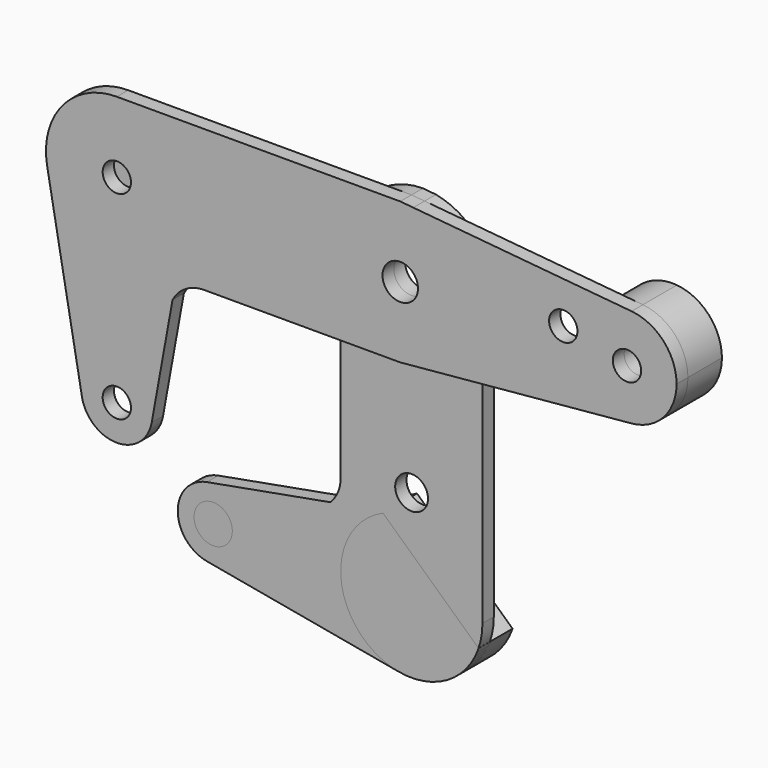
from build123d import *

# Parameters (mm, degrees)
F0_R     = 3.175
F0_R_2   = 3.9751
F2_DEPTH = 3.175
F1_R     = 4.2892452459
F1_R_2   = 3.6765959768
F1_R_3   = 5.1795527056
F3_DEPTH = 3.175
F6_DEPTH = 9.525


with BuildPart() as f2:
    # F0 (on Front) → F2 (new body)
    with BuildSketch(Plane.XZ):
        with BuildLine():
            ThreePointArc((-63.5, 15.875), (-52.2746798487, 11.2253201513), (-47.625, 0))
            ThreePointArc((-47.625, 0), (-62.076859197, -15.8110814069), (-79.1198403471, -2.8348214286))
            Line((-79.1198403471, -2.8348214286), (-71.3099201735, -45.8674107143))
            ThreePointArc((-71.3099201735, -45.8674107143), (-64.2115704015, -36.5444592966), (-55.5625, -44.45))
            ThreePointArc((-55.5625, -44.45), (-55.5944592966, -45.1615704015), (-55.6900798265, -45.8674107143))
            Line((-55.6900798265, -45.8674107143), (-51.0209685693, -20.140650057))
            ThreePointArc((-51.0209685693, -20.140650057), (-48.093941688, -17.0245166153), (-43.976128489, -15.875))
            Line((-43.976128489, -15.875), (0, -15.875))
            ThreePointArc((0, -15.875), (-15.875, 0), (0, 15.875))
            Line((0, 15.875), (-63.5, 15.875))
        make_face()
        with BuildLine():
            Line((51.8269366371, 11.0649472386), (2.9215490166, 15.6038513305))
            ThreePointArc((2.9215490166, 15.6038513305), (12.2146472655, 10.1399219514), (15.875, 0))
            ThreePointArc((15.875, 0), (12.2146472655, -10.1399219514), (2.9215490166, -15.6038513305))
            Line((2.9215490166, -15.6038513305), (51.8269366371, -11.0649472386))
            ThreePointArc((51.8269366371, -11.0649472386), (39.6875, 0), (51.8269366371, 11.0649472386))
        make_face()
        with Locations((36.5252, 3.175)):
            Circle(F0_R, mode=Mode.SUBTRACT)
        with BuildLine():
            Line((2.9215490166, 15.6038513305), (0, 15.875))
            ThreePointArc((0, 15.875), (-15.875, 0), (0, -15.875))
            Line((0, -15.875), (2.9215490166, -15.6038513305))
            ThreePointArc((2.9215490166, -15.6038513305), (12.2146472655, -10.1399219514), (15.875, 0))
            ThreePointArc((15.875, 0), (12.2146472655, 10.1399219514), (2.9215490166, 15.6038513305))
        make_face()
        Circle(F0_R_2, mode=Mode.SUBTRACT)
        with BuildLine():
            ThreePointArc((61.9125, 0), (59.0127793599, 7.4858474093), (51.8269366371, 11.0649472386))
            ThreePointArc((51.8269366371, 11.0649472386), (39.6875, 0), (51.8269366371, -11.0649472386))
            ThreePointArc((51.8269366371, -11.0649472386), (59.0127793599, -7.4858474093), (61.9125, 0))
        make_face()
        with Locations((50.8, 0)):
            Circle(F0_R, mode=Mode.SUBTRACT)
        with BuildLine():
            ThreePointArc((-79.1198403471, -2.8348214286), (-62.076859197, -15.8110814069), (-47.625, 0))
            ThreePointArc((-47.625, 0), (-52.2746798487, 11.2253201513), (-63.5, 15.875))
            ThreePointArc((-63.5, 15.875), (-75.6864353931, 10.1738103683), (-79.1198403471, -2.8348214286))
        make_face()
        with Locations((-63.5, 0)):
            Circle(F0_R, mode=Mode.SUBTRACT)
        with BuildLine():
            ThreePointArc((-55.5625, -44.45), (-64.2115704015, -36.5444592966), (-71.3099201735, -45.8674107143))
            ThreePointArc((-71.3099201735, -45.8674107143), (-63.5, -52.3875), (-55.6900798265, -45.8674107143))
            ThreePointArc((-55.6900798265, -45.8674107143), (-55.5944592966, -45.1615704015), (-55.5625, -44.45))
        make_face()
        with Locations((-63.5, -44.45)):
            Circle(F0_R, mode=Mode.SUBTRACT)
    extrude(amount=F2_DEPTH)


with BuildPart() as f3:
    # F1 (on Front) → F3 (new body)
    with BuildSketch(Plane.XZ):
        with BuildLine():
            ThreePointArc((-45.8674107143, -55.6900798265), (-52.3875, -63.5), (-45.8674107143, -71.3099201735))
            ThreePointArc((-45.8674107143, -71.3099201735), (-39.3630948158, -69.5932176965), (-36.5125, -63.5))
            ThreePointArc((-36.5125, -63.5), (-39.3630948158, -57.4067823035), (-45.8674107143, -55.6900798265))
        make_face()
        with Locations((-44.45, -63.5)):
            Circle(F1_R, mode=Mode.SUBTRACT)
        with BuildLine():
            ThreePointArc((-2.8348214286, -79.1198403471), (-10.1738103683, -51.3135646069), (15.875, -63.5))
            Line((15.875, -63.5), (15.875, 0))
            ThreePointArc((15.875, 0), (0, -15.875), (-15.875, 0))
            Line((-15.875, 0), (-15.875, -45.0455299837))
            ThreePointArc((-15.875, -45.0455299837), (-16.4809135011, -48.0897270637), (-18.2062962849, -50.6699056006))
            Line((-18.2062962849, -50.6699056006), (-45.8674107143, -55.6900798265))
            ThreePointArc((-45.8674107143, -55.6900798265), (-39.3630948158, -57.4067823035), (-36.5125, -63.5))
            ThreePointArc((-36.5125, -63.5), (-39.3630948158, -69.5932176965), (-45.8674107143, -71.3099201735))
            Line((-45.8674107143, -71.3099201735), (-2.8348214286, -79.1198403471))
        make_face()
        with Locations((0, -42.8498)):
            Circle(F1_R_2, mode=Mode.SUBTRACT)
        with BuildLine():
            ThreePointArc((-2.8348214286, -79.1198403471), (10.1738103683, -75.6864353931), (15.875, -63.5))
            ThreePointArc((15.875, -63.5), (-10.1738103683, -51.3135646069), (-2.8348214286, -79.1198403471))
        make_face()
        with Locations((0, -63.5)):
            Circle(F1_R_3, mode=Mode.SUBTRACT)
    extrude(amount=-F3_DEPTH)

    # F0 (on Front) → F3, piece 2 (join)
    with BuildSketch(Plane.XZ):
        with BuildLine():
            Line((2.9215490166, 15.6038513305), (0, 15.875))
            ThreePointArc((0, 15.875), (-15.875, 0), (0, -15.875))
            Line((0, -15.875), (2.9215490166, -15.6038513305))
            ThreePointArc((2.9215490166, -15.6038513305), (12.2146472655, -10.1399219514), (15.875, 0))
            ThreePointArc((15.875, 0), (12.2146472655, 10.1399219514), (2.9215490166, 15.6038513305))
        make_face()
        Circle(F0_R_2, mode=Mode.SUBTRACT)
    extrude(amount=-F3_DEPTH)


with BuildPart() as f6:
    # F4 (on face) → F6 (new body, through all)
    with BuildSketch(Plane.XZ):
        with BuildLine():
            Line((15.0065312392, -68.678768692), (-6.4073053166, -48.9754668378))
            ThreePointArc((-6.4073053166, -48.9754668378), (-15.7646769793, -65.3683106647), (-2.8348214286, -79.1198403471))
            ThreePointArc((-2.8348214286, -79.1198403471), (8.0182058002, -77.2012408469), (15.0065312392, -68.678768692))
        make_face()
    extrude(amount=-F6_DEPTH)


with BuildPart() as f6b:
    # F1 (on Front) → F6, piece 2 (new body, through all)
    with BuildSketch(Plane.XZ):
        with Locations((-44.45, -63.5)):
            Circle(F1_R)
    extrude(amount=-F6_DEPTH)


with BuildPart() as f6c:
    # F0 (on Front) → F6, piece 3 (new body, through all)
    with BuildSketch(Plane.XZ):
        with Locations((-63.5, 0)):
            Circle(F0_R)
    extrude(amount=-F6_DEPTH)


with BuildPart() as f6d:
    # F0 (on Front) → F6, piece 4 (new body, through all)
    with BuildSketch(Plane.XZ):
        with BuildLine():
            ThreePointArc((61.9125, 0), (59.0127793599, 7.4858474093), (51.8269366371, 11.0649472386))
            ThreePointArc((51.8269366371, 11.0649472386), (39.6875, 0), (51.8269366371, -11.0649472386))
            ThreePointArc((51.8269366371, -11.0649472386), (59.0127793599, -7.4858474093), (61.9125, 0))
        make_face()
        with Locations((50.8, 0)):
            Circle(F0_R, mode=Mode.SUBTRACT)
    extrude(amount=-F6_DEPTH)


solid = Compound([f2.part, f3.part, f6.part, f6b.part, f6c.part, f6d.part])
